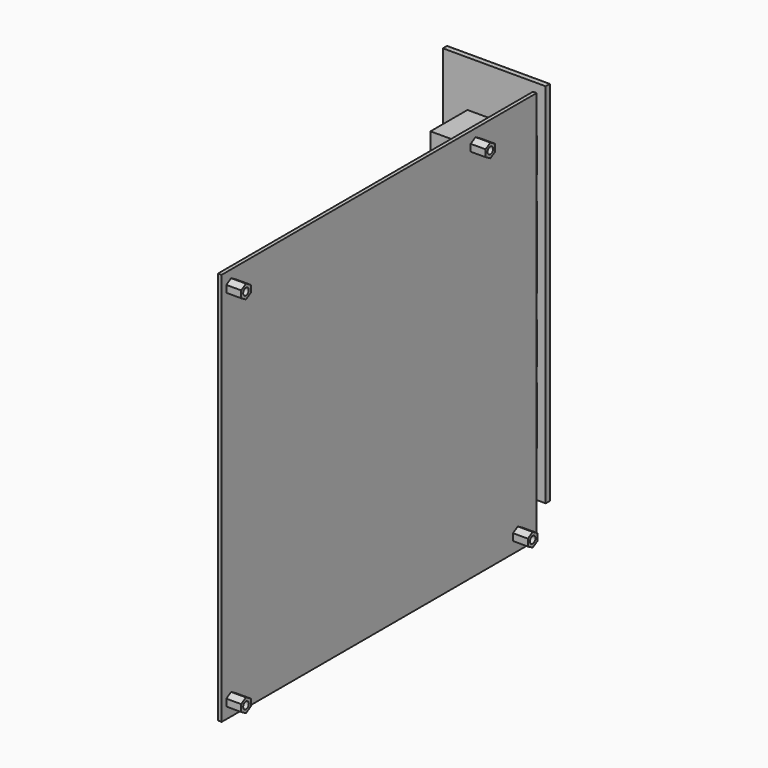
from build123d import *

# Parameters (mm, degrees)
F0_W          = 10.16
F0_H          = 6.35
F0_R          = 1.98
F0_W_2        = 8
F0_H_2        = 1.57
F0_W_3        = 71.65
F0_H_3        = 1.6
F0_W_4        = 11.65
F1_DEPTH      = 1.57
F2_DEPTH      = 11.25
F3_R          = 1.5
F4_DEPTH      = 6.43
F0_W_5        = 0.94
F0_H_4        = 158.75
F5_DEPTH      = 3.81
F5_DEPTH_BACK = 40.64
F6_W          = 44.45
F6_H          = 158.75
F6_W_2        = 40.45
F6_H_2        = 154.75
F7_DEPTH      = 2
F8_R          = 0.99999
F9_W          = 30
F9_H          = 15
F10_DEPTH     = 20
F9_W_2        = 25
F9_H_2        = 35
F11_DEPTH     = 25
F9_H_3        = 18
F12_DEPTH     = 30
F9_W_3        = 38
F9_H_4        = 25
F13_DEPTH     = 23
F14_SIZE      = 5
F15_W         = 4
F15_H         = 1.6
F16_DEPTH     = 2
F17_DEPTH     = 7.9


# Not quite as in the source:
# - a fillet or chamfer is up to 0.001 mm smaller than in the source, because OpenCascade refuses the exact size


with BuildPart() as f1:
    # F0 (on Right) → F1 (new body)
    with BuildSketch(Plane.YZ):
        with Locations((5.08, 206.375)):
            Rectangle(F0_W, F0_H)
        with BuildLine():
            Line((0, 203.2), (0, 209.55))
            Line((0, 209.55), (-22.86, 209.55))
            Line((-22.86, 209.55), (-22.86, 205.18))
            ThreePointArc((-22.86, 205.18), (-21.4599285733, 204.6000714267), (-20.88, 203.2))
            Line((-20.88, 203.2), (0, 203.2))
        make_face()
        with BuildLine():
            Line((-22.86, 205.18), (-22.86, 209.55))
            Line((-22.86, 209.55), (-154.94, 209.55))
            Line((-154.94, 209.55), (-154.94, 205.18))
            ThreePointArc((-154.94, 205.18), (-153.5399285733, 204.6000714267), (-152.96, 203.2))
            Line((-152.96, 203.2), (-24.84, 203.2))
            ThreePointArc((-24.84, 203.2), (-24.2600714267, 204.6000714267), (-22.86, 205.18))
        make_face()
        with BuildLine():
            Line((-154.94, 205.18), (-154.94, 209.55))
            Line((-154.94, 209.55), (-160.02, 209.55))
            Line((-160.02, 209.55), (-160.02, 203.2))
            Line((-160.02, 203.2), (-156.92, 203.2))
            ThreePointArc((-156.92, 203.2), (-156.3400714267, 204.6000714267), (-154.94, 205.18))
        make_face()
        with BuildLine():
            Line((0, 47.7), (0, 203.2))
            Line((0, 203.2), (-20.88, 203.2))
            ThreePointArc((-20.88, 203.2), (-22.86, 201.22), (-24.84, 203.2))
            Line((-24.84, 203.2), (-152.96, 203.2))
            ThreePointArc((-152.96, 203.2), (-154.94, 201.22), (-156.92, 203.2))
            Line((-156.92, 203.2), (-160.02, 203.2))
            Line((-160.02, 203.2), (-160.02, 39.37))
            Line((-160.02, 39.37), (0, 39.37))
            Line((0, 39.37), (0, 43.74))
            ThreePointArc((0, 43.74), (-1.98, 45.72), (0, 47.7))
        make_face()
        with Locations((-154.94, 45.72)):
            Circle(F0_R, mode=Mode.SUBTRACT)
        Polygon((-121.44, 51.04), (-46.94, 51.04), (-32.44, 51.04), (-32.44, 43.54), (-46.94, 43.54), (-121.44, 43.54), align=None, mode=Mode.SUBTRACT)
        with Locations((-27.14, 47.29)):
            Rectangle(F0_W_2, F0_H_2, mode=Mode.SUBTRACT)
        with BuildLine():
            Line((10.16, 45.72), (10.16, 203.2))
            Line((10.16, 203.2), (0, 203.2))
            Line((0, 203.2), (0, 47.7))
            ThreePointArc((0, 47.7), (1.4000714267, 47.1200714267), (1.98, 45.72))
            Line((1.98, 45.72), (10.16, 45.72))
        make_face()
        with BuildLine():
            Line((10.16, 39.37), (10.16, 45.72))
            Line((10.16, 45.72), (1.98, 45.72))
            ThreePointArc((1.98, 45.72), (1.4000714267, 44.3199285733), (0, 43.74))
            Line((0, 43.74), (0, 39.37))
            Line((0, 39.37), (10.16, 39.37))
        make_face()
        Polygon((-32.44, 51.04), (-46.94, 51.04), (-121.44, 51.04), (-121.44, 43.54), (-46.94, 43.54), (-32.44, 43.54), align=None)
        with Locations((-83.615, 47.29)):
            Rectangle(F0_W_3, F0_H_3, mode=Mode.SUBTRACT)
        with Locations((-40.265, 47.29)):
            Rectangle(F0_W_4, F0_H_3, mode=Mode.SUBTRACT)
        with Locations((-40.265, 47.29)):
            Rectangle(F0_W_4, F0_H_3)
        with Locations((-83.615, 47.29)):
            Rectangle(F0_W_3, F0_H_3)
        with Locations((-27.14, 47.29)):
            Rectangle(F0_W_2, F0_H_2)
    extrude(amount=F1_DEPTH)

    # F0 (on Right) → F2 (join)
    with BuildSketch(Plane.YZ):
        Polygon((-32.44, 51.04), (-46.94, 51.04), (-121.44, 51.04), (-121.44, 43.54), (-46.94, 43.54), (-32.44, 43.54), align=None)
        with Locations((-83.615, 47.29)):
            Rectangle(F0_W_3, F0_H_3, mode=Mode.SUBTRACT)
        with Locations((-40.265, 47.29)):
            Rectangle(F0_W_4, F0_H_3, mode=Mode.SUBTRACT)
    extrude(amount=-F2_DEPTH)

    # F3 (on face) → F4 (join)
    with BuildSketch(Plane.YZ.offset(1.57)):
        Polygon((-154.94, 200.2), (-152.3419237886, 201.7), (-152.3419237886, 204.7), (-154.94, 206.2), (-157.5380762114, 204.7), (-157.5380762114, 201.7), align=None)
        with Locations((-154.94, 203.2)):
            Circle(F3_R, mode=Mode.SUBTRACT)
        Polygon((-154.94, 42.72), (-152.3419237886, 44.22), (-152.3419237886, 47.22), (-154.94, 48.72), (-157.5380762114, 47.22), (-157.5380762114, 44.22), align=None)
        with Locations((-154.94, 45.72)):
            Circle(F3_R, mode=Mode.SUBTRACT)
        Polygon((0, 42.72), (2.5980762114, 44.22), (2.5980762114, 47.22), (0, 48.72), (-2.5980762114, 47.22), (-2.5980762114, 44.22), align=None)
        with Locations((0, 45.72)):
            Circle(F3_R, mode=Mode.SUBTRACT)
        Polygon((-22.86, 200.2), (-20.2619237886, 201.7), (-20.2619237886, 204.7), (-22.86, 206.2), (-25.4580762114, 204.7), (-25.4580762114, 201.7), align=None)
        with Locations((-22.86, 203.2)):
            Circle(F3_R, mode=Mode.SUBTRACT)
    extrude(amount=F4_DEPTH)



with BuildPart() as f5:
    # F0 (on Right) → F5 (new body, two sides)
    with BuildSketch(Plane.YZ) as f5_sk:
        with Locations((12.74, 132.615)):
            Rectangle(F0_W_5, F0_H_4)
    extrude(amount=F5_DEPTH)
    extrude(f5_sk.sketch, amount=-F5_DEPTH_BACK)

    # F6 (on face) → F7 (join)
    with BuildSketch(Plane(origin=(0, 13.21, 0), x_dir=(-1, 0, 0), z_dir=(0, 1, 0))):
        with Locations((18.415, 132.615)):
            Rectangle(F6_W, F6_H)
        with Locations((18.415, 132.615)):
            Rectangle(F6_W_2, F6_H_2, mode=Mode.SUBTRACT)
    extrude(amount=F7_DEPTH)

    # F8 (radius 1 in the source; OpenCascade refuses exactly that, so slightly less here)
    f8_edges = [f5.edges().sort_by_distance(p)[0] for p in [
        (1.81, 15.21, 132.615),
        (-18.415, 15.21, 209.99),
        (-38.64, 15.21, 132.615),
        (-18.415, 15.21, 55.24),
        (-18.415, 15.21, 53.24),
        (-40.64, 15.21, 132.615),
        (3.81, 15.21, 132.615),
        (-18.415, 15.21, 211.99),
    ]]
    fillet(f8_edges, radius=F8_R)


with BuildPart() as f1_1:
    add(f1.part)

    add(f5.part)  # F10 merges F5
    # F9 (on face) → F10 (join)
    with BuildSketch(Plane.XZ.offset(-12.27)):
        with Locations((-15, 184.49)):
            Rectangle(F9_W, F9_H)
    extrude(amount=F10_DEPTH)

    # F9 (on face) → F11 (join)
    with BuildSketch(Plane.XZ.offset(-12.27)):
        with Locations((-12.5, 149.49)):
            Rectangle(F9_W_2, F9_H_2)
    extrude(amount=F11_DEPTH)

    # F9 (on face) → F12 (join)
    with BuildSketch(Plane.XZ.offset(-12.27)):
        with Locations((-15, 112.99)):
            Rectangle(F9_W, F9_H_3)
    extrude(amount=F12_DEPTH)

    # F9 (on face) → F13 (join)
    with BuildSketch(Plane.XZ.offset(-12.27)):
        with Locations((-19, 85.49)):
            Rectangle(F9_W_3, F9_H_4)
    extrude(amount=F13_DEPTH)

    # F14
    f14_edges = [f1_1.edges().sort_by_distance(p)[0] for p in [
        (-25, -12.73, 149.49),
    ]]
    chamfer(f14_edges, length=F14_SIZE)

    # F15 (on face) → F16 (cut)
    with BuildSketch(Plane(origin=(0, -46.09, 0), x_dir=(-1, 0, 0), z_dir=(0, 1, 0))):
        with Locations((2, 47.29)):
            Rectangle(F15_W, F15_H)
    extrude(amount=-F16_DEPTH, mode=Mode.SUBTRACT)

    # F0 (on Right) → F17 (join)
    with BuildSketch(Plane.YZ):
        with Locations((-27.14, 47.29)):
            Rectangle(F0_W_2, F0_H_2)
    extrude(amount=-F17_DEPTH)


solid = f1_1.part
